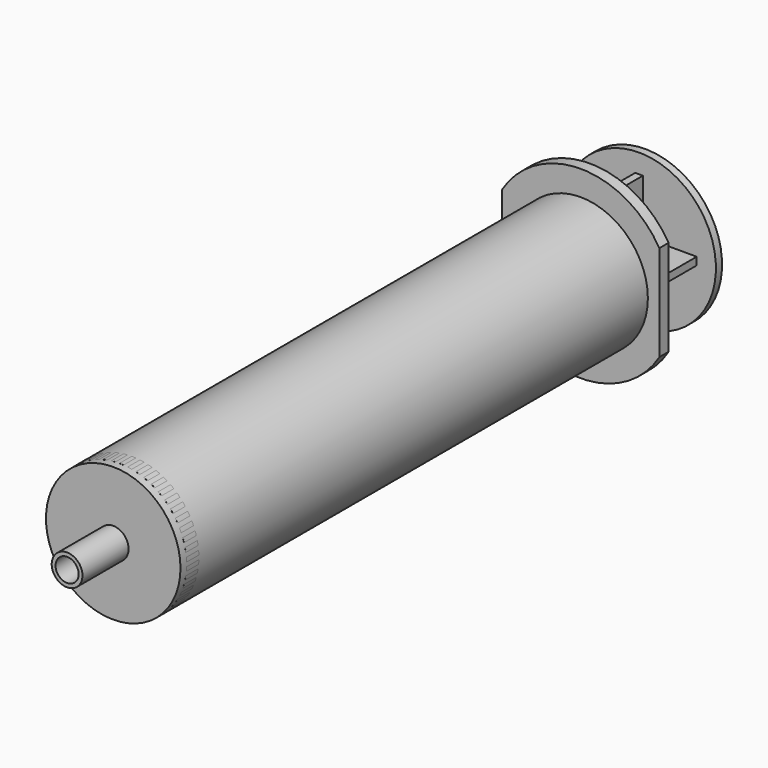
from build123d import *

# Parameters (mm, degrees)
F0_R      = 17.5
F0_R_2    = 16.5
F1_DEPTH  = 150
F2_R      = 17.5
F3_DEPTH  = 2
F4_R      = 4
F5_DEPTH  = 15
F6_R      = 3
F7_DEPTH  = 17
F8_R      = 17.5
F8_R_2    = 16.5
F9_DEPTH  = 3
F10_R     = 17.5
F11_DEPTH = 4
F12_W     = 14
F12_H     = 2
F12_W_2   = 2
F12_H_2   = 14
F13_DEPTH = 165
F14_R     = 20
F15_DEPTH = 2


with BuildPart() as f1:
    # F0 (on Front) → F1 (new body)
    with BuildSketch(Plane.XZ):
        Circle(F0_R)
        Circle(F0_R_2, mode=Mode.SUBTRACT)
    extrude(amount=F1_DEPTH)

    # F2 (on face) → F3 (join)
    with BuildSketch(Plane.XZ.offset(150)):
        Circle(F2_R)
    extrude(amount=F3_DEPTH)

    # F4 (on face) → F5 (join)
    with BuildSketch(Plane.XZ.offset(152)):
        Circle(F4_R)
    extrude(amount=F5_DEPTH)

    # F6 (on face) → F7 (cut, through all)
    with BuildSketch(Plane.XZ.offset(167)):
        Circle(F6_R)
    extrude(amount=-F7_DEPTH, mode=Mode.SUBTRACT)

    # F8 (on face) → F9 (join)
    with BuildSketch(Plane(origin=(0, 0, 0), x_dir=(-1, 0, 0), z_dir=(0, 1, 0))):
        with BuildLine():
            Line((20.5, -12.4799839743), (20.5, 12.4799839743))
            ThreePointArc((20.5, 12.4799839743), (0, 24), (-20.5, 12.4799839743))
            Line((-20.5, 12.4799839743), (-20.5, -12.4799839743))
            ThreePointArc((-20.5, -12.4799839743), (0, -24), (20.5, -12.4799839743))
        make_face()
        Circle(F8_R, mode=Mode.SUBTRACT)
        Circle(F8_R)
        Circle(F8_R_2, mode=Mode.SUBTRACT)
    extrude(amount=F9_DEPTH)


with BuildPart() as f11:
    # F10 (on face) → F11 (new body)
    with BuildSketch(Plane(origin=(0, -150, 0), x_dir=(-1, 0, 0), z_dir=(0, 1, 0))):
        Circle(F10_R)
    extrude(amount=F11_DEPTH)

    # F12 (on face) → F13 (join)
    with BuildSketch(Plane(origin=(0, -146, 0), x_dir=(-1, 0, 0), z_dir=(0, 1, 0))):
        with Locations((8, 0)):
            Rectangle(F12_W, F12_H)
        Rectangle(F12_W_2, F12_H)
        with Locations((0, 8)):
            Rectangle(F12_W_2, F12_H_2)
        with Locations((-8, 0)):
            Rectangle(F12_W, F12_H)
        with Locations((0, -8)):
            Rectangle(F12_W_2, F12_H_2)
    extrude(amount=F13_DEPTH)

    # F14 (on face) → F15 (join)
    with BuildSketch(Plane(origin=(0, 19, 0), x_dir=(-1, 0, 0), z_dir=(0, 1, 0))):
        Circle(F14_R)
    extrude(amount=F15_DEPTH)


solid = Compound([f1.part, f11.part])
